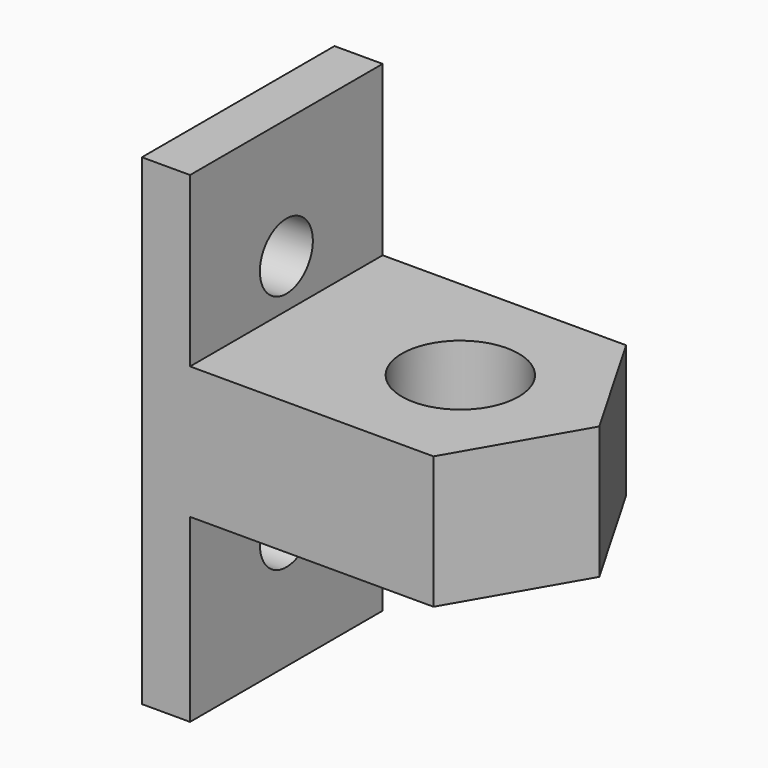
from build123d import *

# Parameters (mm, degrees)
F0_R     = 4.85
F1_DEPTH = 11
F2_W     = 20
F2_H     = 40
F3_DEPTH = 4
F4_W     = 9
F4_H     = 40
F5_DEPTH = 1.5
F6_SIZE  = 1.49999
F7_R     = 2.75
F8_DEPTH = 31.501


# Not quite as in the source:
# - a fillet or chamfer is up to 0.001 mm smaller than in the source, because OpenCascade refuses the exact size


with BuildPart() as f1:
    # F0 (on Top) → F1 (new body)
    with BuildSketch(Plane.XY):
        Polygon((5.7735026919, 10), (-5.7735026919, 10), (-14.4529946162, 10), (-14.4529946162, -10), (-5.7735026919, -10), (5.7735026919, -10), (11.5470053838, 0), align=None)
        Circle(F0_R, mode=Mode.SUBTRACT)
    extrude(amount=F1_DEPTH)

    # F2 (on face) → F3 (join)
    with BuildSketch(Plane(origin=(-14.4529946162, 0, 0), x_dir=(0, -1, 0), z_dir=(-1, 0, 0))):
        with Locations((0, 5)):
            Rectangle(F2_W, F2_H)
    extrude(amount=F3_DEPTH)

    # F4 (on face) → F5 (join)
    with BuildSketch(Plane(origin=(-18.4529946162, 0, 0), x_dir=(0, -1, 0), z_dir=(-1, 0, 0))):
        with Locations((0, 5)):
            Rectangle(F4_W, F4_H)
    extrude(amount=F5_DEPTH)

    # F6 (size 1.5 in the source; OpenCascade refuses exactly that, so slightly less here)
    f6_edges = [f1.edges().sort_by_distance(p)[0] for p in [
        (-19.952995, 0, 25),
        (-19.952995, 4.5, 5),
        (-19.952995, 0, -15),
        (-19.952995, -4.5, 5),
    ]]
    chamfer(f6_edges, length=F6_SIZE)

    # F7 (on face) → F8 (cut, through all)
    with BuildSketch(Plane(origin=(-19.9529946162, 0, 0), x_dir=(0, -1, 0), z_dir=(-1, 0, 0))):
        with Locations((0, 15)):
            Circle(F7_R)
        with Locations((0, -5)):
            Circle(F7_R)
    extrude(amount=-F8_DEPTH, mode=Mode.SUBTRACT)


solid = f1.part
